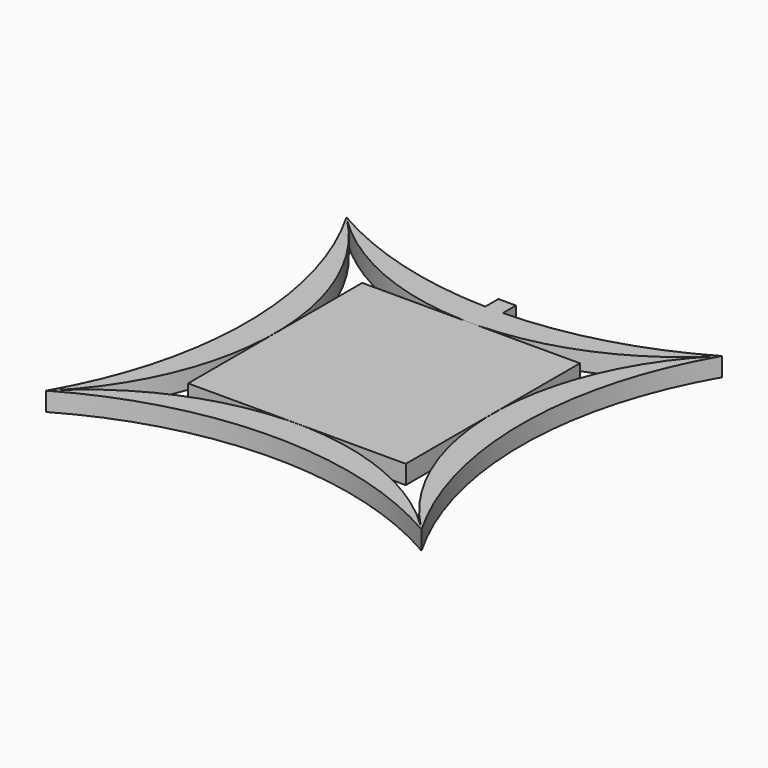
from build123d import *

# Parameters (mm, degrees)
F1_DEPTH = 5
F3_DEPTH = 100
F4_T     = -2


# Not quite as in the source:
# - a feature names something its author has since deleted; it is built from what else it names


with BuildPart() as f1:
    # F0 (on Top) → F1 (new body)
    with BuildSketch(Plane.XY):
        with BuildLine():
            ThreePointArc((48.9897948557, -48.9897948557), (49.4974746831, -49.4923201726), (50, -50))
            ThreePointArc((50, -50), (36.6025403784, 0), (50, 50))
            ThreePointArc((50, 50), (49.4974746831, 49.4923201726), (48.9897948557, 48.9897948557))
            ThreePointArc((48.9897948557, 48.9897948557), (34.1823878716, 26.4575131106), (28.9897948557, 0))
            ThreePointArc((28.9897948557, 0), (34.1823878716, -26.4575131106), (48.9897948557, -48.9897948557))
        make_face()
    extrude(amount=F1_DEPTH)


with BuildPart() as f1b:
    # F0 (on Top) → F1, piece 2 (new body)
    with BuildSketch(Plane.XY):
        with BuildLine():
            ThreePointArc((-50, -50), (0, -36.6025403784), (50, -50))
            ThreePointArc((50, -50), (49.4923201726, -49.4974746831), (48.9897948557, -48.9897948557))
            ThreePointArc((48.9897948557, -48.9897948557), (26.4575131106, -34.1823878716), (0, -28.9897948557))
            ThreePointArc((0, -28.9897948557), (-26.4575131106, -34.1823878716), (-48.9897948557, -48.9897948557))
            ThreePointArc((-48.9897948557, -48.9897948557), (-49.4923201726, -49.4974746831), (-50, -50))
        make_face()
    extrude(amount=F1_DEPTH)


with BuildPart() as f1c:
    # F0 (on Top) → F1, piece 3 (new body)
    with BuildSketch(Plane.XY):
        with BuildLine():
            ThreePointArc((-50, 50), (-36.6025403784, 0), (-50, -50))
            ThreePointArc((-50, -50), (-49.4974746831, -49.4923201726), (-48.9897948557, -48.9897948557))
            ThreePointArc((-48.9897948557, -48.9897948557), (-34.1823878716, -26.4575131106), (-28.9897948557, 0))
            ThreePointArc((-28.9897948557, 0), (-34.1823878716, 26.4575131106), (-48.9897948557, 48.9897948557))
            ThreePointArc((-48.9897948557, 48.9897948557), (-49.4974746831, 49.4923201726), (-50, 50))
        make_face()
    extrude(amount=F1_DEPTH)


with BuildPart() as f1d:
    # F0 (on Top) → F1, piece 4 (new body)
    with BuildSketch(Plane.XY):
        with BuildLine():
            ThreePointArc((48.9897948557, 48.9897948557), (49.4923201726, 49.4974746831), (50, 50))
            ThreePointArc((50, 50), (27.0079233825, 40.318730345), (2.3349747062, 36.6298046295))
            Line((2.3349747062, 36.6298046295), (2.3349747062, 29.0287493152))
            ThreePointArc((2.3349747062, 29.0287493152), (27.534865669, 34.6327348499), (48.9897948557, 48.9897948557))
        make_face()
        with BuildLine():
            ThreePointArc((-2.3349747062, 36.6298046295), (-27.0079233825, 40.318730345), (-50, 50))
            ThreePointArc((-50, 50), (-49.4923201726, 49.4974746831), (-48.9897948557, 48.9897948557))
            ThreePointArc((-48.9897948557, 48.9897948557), (-27.534865669, 34.6327348499), (-2.3349747062, 29.0287493152))
            Line((-2.3349747062, 29.0287493152), (-2.3349747062, 36.6298046295))
        make_face()
        with BuildLine():
            Line((2.3349747062, 29.0287493152), (2.3349747062, 36.6298046295))
            ThreePointArc((2.3349747062, 36.6298046295), (0, 36.6025403784), (-2.3349747062, 36.6298046295))
            Line((-2.3349747062, 36.6298046295), (-2.3349747062, 29.0287493152))
            ThreePointArc((-2.3349747062, 29.0287493152), (-1.1676498114, 28.9995341481), (0, 28.9897948557))
            ThreePointArc((0, 28.9897948557), (1.1676498114, 28.9995341481), (2.3349747062, 29.0287493152))
        make_face()
        with BuildLine():
            ThreePointArc((-2.3349747062, 36.6298046295), (0, 36.6025403784), (2.3349747062, 36.6298046295))
            Line((2.3349747062, 36.6298046295), (2.3349747062, 40.9987472145))
            Line((2.3349747062, 40.9987472145), (-2.3349747062, 40.9987472145))
            Line((-2.3349747062, 40.9987472145), (-2.3349747062, 36.6298046295))
        make_face()
    extrude(amount=F1_DEPTH)

    # F2 (on face) → F3 (cut)
    with BuildSketch(Plane(origin=(0, 40.9987472145, 0), x_dir=(-1, 0, 0), z_dir=(0, 1, 0))):
        with BuildLine():
            ThreePointArc((1.7021905713, 2.5), (1.2036304958, 3.7036304958), (0, 4.2021905713))
            Line((0, 4.2021905713), (0, 0.7978094287))
            ThreePointArc((0, 0.7978094287), (1.2036304958, 1.2963695042), (1.7021905713, 2.5))
        make_face()
        with BuildLine():
            Line((0, 0.7978094287), (0, 4.2021905713))
            ThreePointArc((0, 4.2021905713), (-1.7021905713, 2.5), (0, 0.7978094287))
        make_face()
    extrude(amount=-F3_DEPTH, mode=Mode.SUBTRACT)


with BuildPart() as f1e:
    # F0 (on Top) → F1, piece 5 (new body)
    with BuildSketch(Plane.XY):
        Polygon((-28.9897948557, -28.9897948557), (0, -28.9897948557), (28.9897948557, -28.9897948557), (28.9897948557, 0), (28.9897948557, 28.9897948557), (2.3349747062, 28.9897948557), (0, 28.9897948557), (-2.3349747062, 28.9897948557), (-28.9897948557, 28.9897948557), (-28.9897948557, 0), align=None)
    extrude(amount=F1_DEPTH)

    # F4
    f4_openings = [f1e.faces().sort_by_distance(p)[0] for p in [
        (0, 0, 0),
    ]]
    offset(amount=F4_T, openings=f4_openings)


solid = Compound([f1.part, f1b.part, f1c.part, f1d.part, f1e.part])
